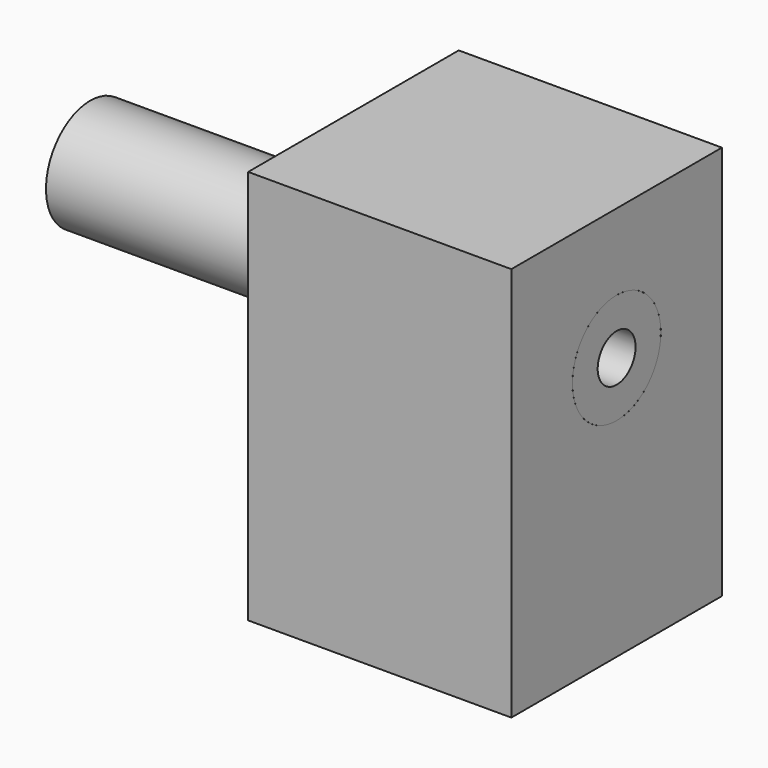
from build123d import *

# Parameters (mm, degrees)
F0_R      = 2.667
F0_R_2    = 1.143
F1_DEPTH  = 12.7
F3_R      = 0.889
F5_W      = 12.7
F5_H      = 19.05
F6_DEPTH  = 12.7
F7_R      = 2.667
F8_DEPTH  = 12.701
F9_R      = 4.4196
F10_DEPTH = 1.778
F11_R     = 5.08
F12_DEPTH = 0.508
F13_SIZE  = 0.254
F14_R     = 2.667
F14_R_2   = 1.143
F15_DEPTH = 12.7


with BuildPart() as f1:
    # F0 (on Right) → F1 (new body)
    with BuildSketch(Plane.YZ):
        Circle(F0_R)
        Circle(F0_R_2, mode=Mode.SUBTRACT)
    extrude(amount=F1_DEPTH)

    # F14 (on face) → F15 (join)
    with BuildSketch(Plane.YZ.offset(12.7)):
        Circle(F14_R)
        Circle(F14_R_2, mode=Mode.SUBTRACT)
    extrude(amount=F15_DEPTH)


with BuildPart() as f4:
    # F3 (on Front) → F4 (revolve)
    with BuildSketch(Plane.XZ):
        with Locations((13.716, 3.5306)):
            Circle(F3_R)
    revolve(axis=Axis((18.1991, 0, 0), (1, 0, 0)))


with BuildPart() as f6:
    # F5 (on face) → F6 (new body)
    with BuildSketch(Plane.YZ.offset(12.7)):
        with Locations((0, -3.175)):
            Rectangle(F5_W, F5_H)
    extrude(amount=F6_DEPTH)

    # F7 (on face) → F8 (cut, through all)
    with BuildSketch(Plane(origin=(12.7, 0, 0), x_dir=(0, -1, 0), z_dir=(-1, 0, 0))):
        Circle(F7_R)
    extrude(amount=-F8_DEPTH, mode=Mode.SUBTRACT)

    # F9 (on face) → F10 (cut)
    with BuildSketch(Plane(origin=(12.7, 0, 0), x_dir=(0, -1, 0), z_dir=(-1, 0, 0))):
        Circle(F9_R)
    extrude(amount=-F10_DEPTH, mode=Mode.SUBTRACT)

    # F11 (on face) → F12 (cut)
    with BuildSketch(Plane(origin=(12.7, 0, 0), x_dir=(0, -1, 0), z_dir=(-1, 0, 0))):
        Circle(F11_R)
    extrude(amount=-F12_DEPTH, mode=Mode.SUBTRACT)

    # F13
    f13_edges = [f6.edges().sort_by_distance(p)[0] for p in [
        (12.7, 5.08, 0),
        (13.208, 4.4196, 0),
    ]]
    chamfer(f13_edges, length=F13_SIZE)


solid = Compound([f1.part, f4.part, f6.part])
